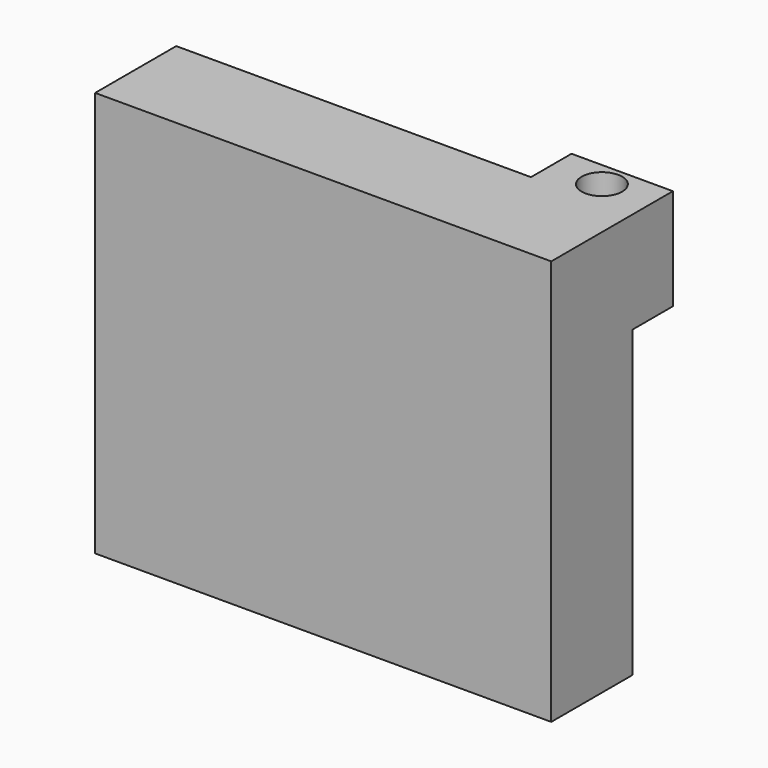
from build123d import *

# Parameters (mm, degrees)
F0_W     = 114.3
F0_H     = 101.6
F1_DEPTH = 25.4
F2_W     = 25.4
F2_H     = 12.7
F3_DEPTH = 25.4
F7_D     = 10.16


# Not quite as in the source:
# - a feature of the source that left no trace in its solid (it failed there, or was rolled back) is left out


with BuildPart() as f1:
    # F0 (on Front) → F1 (new body)
    with BuildSketch(Plane.XZ):
        with Locations((-44.2425758362, 44.6146523613)):
            Rectangle(F0_W, F0_H)
    extrude(amount=F1_DEPTH)

    # F2 (on face) → F3 (join)
    with BuildSketch(Plane.XY.offset(95.4146523613)):
        with Locations((0.2074241638, 6.35)):
            Rectangle(F2_W, F2_H)
    extrude(amount=-F3_DEPTH)

    # F5: union 

    # F7 (through all)
    with Locations(Plane.XY.offset(95.4146523613)):
        with Locations((0.2074241638, 6.35)):
            Hole(F7_D / 2)


solid = f1.part
